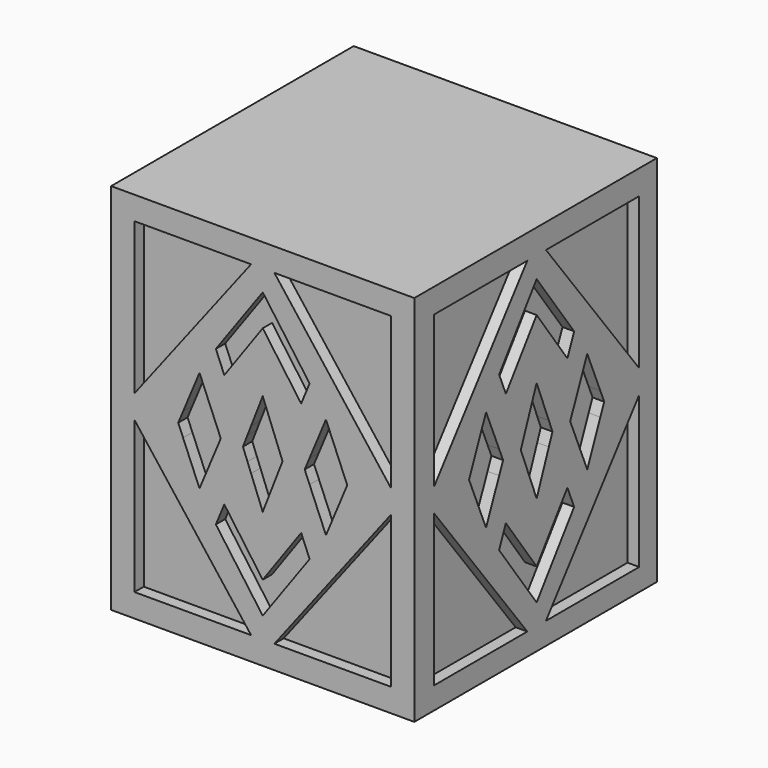
from build123d import *

# Parameters (mm, degrees)
F0_W     = 130
F0_H     = 130
F1_DEPTH = 160
F2_W     = 5
F2_H     = 5.0000008941
F2_H_2   = 5
F3_DEPTH = 5
F4_W     = 5
F4_H     = 5.0000008941
F4_H_2   = 5
F5_DEPTH = 5
F6_W     = 5
F6_H     = 5.0000008941
F6_H_2   = 5
F7_DEPTH = 5
F8_W     = 5
F8_H     = 5.0000008941
F8_H_2   = 5
F9_DEPTH = 5


# Not quite as in the source:
# - ends of sketch curves that miss each other by under 0.0002 mm in the source are joined


with BuildPart() as f1:
    # F0 (on Top) → F1 (new body)
    with BuildSketch(Plane.XY):
        with Locations((65, 65)):
            Rectangle(F0_W, F0_H)
    extrude(amount=F1_DEPTH)

    # F2 (on face) → F3 (cut)
    with BuildSketch(Plane.XZ):
        Polygon((85.1000148058, 113.1451874971), (65, 141.0418897867), (44.8999851942, 113.1451874971), (48.5190190375, 104.3991968036), (65, 127.470523119), (81.4809809625, 104.3991968036), align=None)
        Polygon((44.8999851942, 46.8548125029), (65, 18.9581102133), (85.1000148058, 46.8548125029), (81.4809809625, 55.6008031964), (65, 32.529476881), (48.5190190375, 55.6008031964), align=None)
        Polygon((120, 74.9999991059), (70, 10), (120, 10), align=None)
        Polygon((10, 74.999999702), (10, 10), (60, 10), align=None)
        Polygon((10, 150), (10, 85.0000008941), (60, 150), align=None)
        Polygon((120, 150), (70, 150), (120, 85.0000008941), align=None)
        Polygon((92.1118893847, 85.0000008941), (99.1458630462, 85.0000008941), (92.1118893847, 101.8357127905), align=None)
        Polygon((85.0779157232, 85.0000008941), (92.1118893847, 85.0000008941), (92.1118893847, 101.8357127905), align=None)
        Polygon((82.9889114201, 80), (92.1118893847, 80), (92.1118893847, 85.0000008941), (85.0779157232, 85.0000008941), align=None)
        Polygon((92.1118893847, 80), (101.2348673493, 80), (99.1458630462, 85.0000008941), (92.1118893847, 85.0000008941), align=None)
        Polygon((92.1118893847, 75), (99.1458634198, 75), (101.2348673493, 80), (92.1118893847, 80), align=None)
        Polygon((85.0779153496, 75), (92.1118893847, 75), (92.1118893847, 80), (82.9889114201, 80), align=None)
        Polygon((92.1118893847, 58.1642872095), (92.1118893847, 75), (85.0779153496, 75), align=None)
        Polygon((92.1118893847, 58.1642872095), (99.1458634198, 75), (92.1118893847, 75), align=None)
        Polygon((65, 101.8357127905), (65, 85.0000008941), (71.545128511, 85.0000008941), align=None)
        Polygon((60, 88.9744589067), (60, 85.0000008941), (65, 85.0000008941), (65, 101.8357127905), align=None)
        Polygon((60, 88.9744589067), (58.454871489, 85.0000008941), (60, 85.0000008941), align=None)
        Polygon((58.454871489, 85.0000008941), (56.5110482275, 80), (60, 80), (60, 85.0000008941), align=None)
        Polygon((56.5110482275, 80), (58.4548711414, 75), (60, 75), (60, 80), align=None)
        with Locations((62.5, 82.500000447)):
            Rectangle(F2_W, F2_H)
        with Locations((62.5, 77.5)):
            Rectangle(F2_W, F2_H_2)
        Polygon((65, 75), (60, 75), (60, 71.0255410933), (65, 58.1642872095), align=None)
        Polygon((71.5451288586, 75), (65, 75), (65, 58.1642872095), align=None)
        Polygon((65, 80), (65, 75), (71.5451288586, 75), (73.4889517725, 80), align=None)
        Polygon((65, 85.0000008941), (65, 80), (73.4889517725, 80), (71.545128511, 85.0000008941), align=None)
        Polygon((37.8881106153, 101.8357127905), (37.8881106153, 85.0000008941), (44.9220842768, 85.0000008941), align=None)
        Polygon((37.8881106153, 101.8357127905), (30.8541369538, 85.0000008941), (37.8881106153, 85.0000008941), align=None)
        Polygon((30.8541369538, 85.0000008941), (28.7651326507, 80), (37.8881106153, 80), (37.8881106153, 85.0000008941), align=None)
        Polygon((37.8881106153, 85.0000008941), (37.8881106153, 80), (47.0110885799, 80), (44.9220842768, 85.0000008941), align=None)
        Polygon((28.7651326507, 80), (30.8541365802, 75), (44.9220846504, 75), (47.0110885799, 80), (37.8881106153, 80), align=None)
        Polygon((44.9220846504, 75), (30.8541365802, 75), (37.8881106153, 58.1642872095), align=None)
        Polygon((60, 75), (58.4548711414, 75), (60, 71.0255410933), align=None)
    extrude(amount=-F3_DEPTH, mode=Mode.SUBTRACT)

    # F4 (on face) → F5 (cut)
    with BuildSketch(Plane.YZ.offset(130)):
        Polygon((85.6616547024, 112.6292116297), (65.5616398966, 140.5259139193), (45.4616250909, 112.6292116297), (49.0806589341, 103.8832209362), (65.5616398966, 126.9545472516), (82.0426208592, 103.8832209362), align=None)
        Polygon((85.6395556198, 84.4840250267), (92.6735292813, 84.4840250267), (92.6735292813, 101.3197369231), align=None)
        Polygon((92.6735292813, 84.4840250267), (99.7075029429, 84.4840250267), (92.6735292813, 101.3197369231), align=None)
        Polygon((92.6735292813, 79.4840241326), (101.7965072459, 79.4840241326), (99.7075029429, 84.4840250267), (92.6735292813, 84.4840250267), align=None)
        Polygon((83.5505513168, 79.4840241326), (92.6735292813, 79.4840241326), (92.6735292813, 84.4840250267), (85.6395556198, 84.4840250267), align=None)
        Polygon((85.6395552463, 74.4840241326), (92.6735292813, 74.4840241326), (92.6735292813, 79.4840241326), (83.5505513168, 79.4840241326), align=None)
        Polygon((92.6735292813, 74.4840241326), (99.7075033164, 74.4840241326), (101.7965072459, 79.4840241326), (92.6735292813, 79.4840241326), align=None)
        Polygon((92.6735292813, 57.6483113421), (99.7075033164, 74.4840241326), (92.6735292813, 74.4840241326), align=None)
        Polygon((92.6735292813, 57.6483113421), (92.6735292813, 74.4840241326), (85.6395552463, 74.4840241326), align=None)
        Polygon((65.5616398966, 101.3197369231), (65.5616398966, 84.4840250267), (72.1067684077, 84.4840250267), align=None)
        Polygon((60.5616398966, 88.4584830393), (60.5616398966, 84.4840250267), (65.5616398966, 84.4840250267), (65.5616398966, 101.3197369231), align=None)
        Polygon((60.5616398966, 88.4584830393), (59.0165113856, 84.4840250267), (60.5616398966, 84.4840250267), align=None)
        Polygon((59.0165113856, 84.4840250267), (57.0726881242, 79.4840241326), (60.5616398966, 79.4840241326), (60.5616398966, 84.4840250267), align=None)
        with Locations((63.0616398966, 81.9840245796)):
            Rectangle(F4_W, F4_H)
        Polygon((65.5616398966, 84.4840250267), (65.5616398966, 79.4840241326), (74.0505916691, 79.4840241326), (72.1067684077, 84.4840250267), align=None)
        Polygon((65.5616398966, 79.4840241326), (65.5616398966, 74.4840241326), (72.1067687553, 74.4840241326), (74.0505916691, 79.4840241326), align=None)
        with Locations((63.0616398966, 76.9840241326)):
            Rectangle(F4_W, F4_H_2)
        Polygon((57.0726881242, 79.4840241326), (59.016511038, 74.4840241326), (60.5616398966, 74.4840241326), (60.5616398966, 79.4840241326), align=None)
        Polygon((60.5616398966, 74.4840241326), (59.016511038, 74.4840241326), (60.5616398966, 70.5095652258), align=None)
        Polygon((65.5616398966, 74.4840241326), (60.5616398966, 74.4840241326), (60.5616398966, 70.5095652258), (65.5616398966, 57.6483113421), align=None)
        Polygon((72.1067687553, 74.4840241326), (65.5616398966, 74.4840241326), (65.5616398966, 57.6483113421), align=None)
        Polygon((38.449750512, 101.3197369231), (38.449750512, 84.4840250267), (45.4837241735, 84.4840250267), align=None)
        Polygon((38.449750512, 101.3197369231), (31.4157768504, 84.4840250267), (38.449750512, 84.4840250267), align=None)
        Polygon((31.4157768504, 84.4840250267), (29.3267725474, 79.4840241326), (38.449750512, 79.4840241326), (38.449750512, 84.4840250267), align=None)
        Polygon((38.449750512, 84.4840250267), (38.449750512, 79.4840241326), (47.5727284765, 79.4840241326), (45.4837241735, 84.4840250267), align=None)
        Polygon((29.3267725474, 79.4840241326), (31.4157764769, 74.4840241326), (45.483724547, 74.4840241326), (47.5727284765, 79.4840241326), (38.449750512, 79.4840241326), align=None)
        Polygon((45.483724547, 74.4840241326), (31.4157764769, 74.4840241326), (38.449750512, 57.6483113421), align=None)
        Polygon((45.4616250909, 46.3388366354), (65.5616398966, 18.4421343459), (85.6616547024, 46.3388366354), (82.0426208592, 55.084827329), (65.5616398966, 32.0135010136), (49.0806589341, 55.084827329), align=None)
        Polygon((10.5616398966, 74.4840238346), (10.5616398966, 9.4840241326), (60.5616398966, 9.4840241326), align=None)
        Polygon((120.5616398966, 74.4840232385), (70.5616398966, 9.4840241326), (120.5616398966, 9.4840241326), align=None)
        Polygon((120.5616398966, 149.4840241326), (70.5616398966, 149.4840241326), (120.5616398966, 84.4840250267), align=None)
        Polygon((10.5616398966, 149.4840241326), (10.5616398966, 84.4840250267), (60.5616398966, 149.4840241326), align=None)
    extrude(amount=-F5_DEPTH, mode=Mode.SUBTRACT)

    # F6 (on face) → F7 (cut)
    with BuildSketch(Plane(origin=(0, 130, 0), x_dir=(-1, 0, 0), z_dir=(0, 1, 0))):
        Polygon((-119.4383601034, 149.4840241326), (-119.4383601034, 84.4840250267), (-69.4383601034, 149.4840241326), align=None)
        Polygon((-9.4383601034, 149.4840241326), (-59.4383601034, 149.4840241326), (-9.4383601034, 84.4840250267), align=None)
        Polygon((-44.3383452976, 112.6292116297), (-64.4383601034, 140.5259139193), (-84.5383749091, 112.6292116297), (-80.9193410659, 103.8832209362), (-64.4383601034, 126.9545472516), (-47.9573791408, 103.8832209362), align=None)
        Polygon((-37.3264707187, 84.4840250267), (-30.2924970571, 84.4840250267), (-37.3264707187, 101.3197369231), align=None)
        Polygon((-44.3604443802, 84.4840250267), (-37.3264707187, 84.4840250267), (-37.3264707187, 101.3197369231), align=None)
        Polygon((-46.4494486832, 79.4840241326), (-37.3264707187, 79.4840241326), (-37.3264707187, 84.4840250267), (-44.3604443802, 84.4840250267), align=None)
        Polygon((-37.3264707187, 79.4840241326), (-28.2034927541, 79.4840241326), (-30.2924970571, 84.4840250267), (-37.3264707187, 84.4840250267), align=None)
        Polygon((-37.3264707187, 74.4840241326), (-30.2924966836, 74.4840241326), (-28.2034927541, 79.4840241326), (-37.3264707187, 79.4840241326), align=None)
        Polygon((-44.3604447537, 74.4840241326), (-37.3264707187, 74.4840241326), (-37.3264707187, 79.4840241326), (-46.4494486832, 79.4840241326), align=None)
        Polygon((-37.3264707187, 57.6483113421), (-37.3264707187, 74.4840241326), (-44.3604447537, 74.4840241326), align=None)
        Polygon((-37.3264707187, 57.6483113421), (-30.2924966836, 74.4840241326), (-37.3264707187, 74.4840241326), align=None)
        Polygon((-64.4383601034, 101.3197369231), (-64.4383601034, 84.4840250267), (-57.8932315923, 84.4840250267), align=None)
        Polygon((-69.4383601034, 88.4584830393), (-69.4383601034, 84.4840250267), (-64.4383601034, 84.4840250267), (-64.4383601034, 101.3197369231), align=None)
        Polygon((-69.4383601034, 88.4584830393), (-70.9834886144, 84.4840250267), (-69.4383601034, 84.4840250267), align=None)
        Polygon((-70.9834886144, 84.4840250267), (-72.9273118758, 79.4840241326), (-69.4383601034, 79.4840241326), (-69.4383601034, 84.4840250267), align=None)
        with Locations((-66.9383601034, 81.9840245796)):
            Rectangle(F6_W, F6_H)
        Polygon((-64.4383601034, 84.4840250267), (-64.4383601034, 79.4840241326), (-55.9494083309, 79.4840241326), (-57.8932315923, 84.4840250267), align=None)
        Polygon((-64.4383601034, 79.4840241326), (-64.4383601034, 74.4840241326), (-57.8932312447, 74.4840241326), (-55.9494083309, 79.4840241326), align=None)
        with Locations((-66.9383601034, 76.9840241326)):
            Rectangle(F6_W, F6_H_2)
        Polygon((-72.9273118758, 79.4840241326), (-70.983488962, 74.4840241326), (-69.4383601034, 74.4840241326), (-69.4383601034, 79.4840241326), align=None)
        Polygon((-69.4383601034, 74.4840241326), (-70.983488962, 74.4840241326), (-69.4383601034, 70.5095652258), align=None)
        Polygon((-64.4383601034, 74.4840241326), (-69.4383601034, 74.4840241326), (-69.4383601034, 70.5095652258), (-64.4383601034, 57.6483113421), align=None)
        Polygon((-57.8932312447, 74.4840241326), (-64.4383601034, 74.4840241326), (-64.4383601034, 57.6483113421), align=None)
        Polygon((-91.550249488, 101.3197369231), (-91.550249488, 84.4840250267), (-84.5162758265, 84.4840250267), align=None)
        Polygon((-91.550249488, 101.3197369231), (-98.5842231496, 84.4840250267), (-91.550249488, 84.4840250267), align=None)
        Polygon((-98.5842231496, 84.4840250267), (-100.6732274526, 79.4840241326), (-91.550249488, 79.4840241326), (-91.550249488, 84.4840250267), align=None)
        Polygon((-91.550249488, 84.4840250267), (-91.550249488, 79.4840241326), (-82.4272715235, 79.4840241326), (-84.5162758265, 84.4840250267), align=None)
        Polygon((-100.6732274526, 79.4840241326), (-98.5842235231, 74.4840241326), (-84.516275453, 74.4840241326), (-82.4272715235, 79.4840241326), (-91.550249488, 79.4840241326), align=None)
        Polygon((-84.516275453, 74.4840241326), (-98.5842235231, 74.4840241326), (-91.550249488, 57.6483113421), align=None)
        Polygon((-84.5383749091, 46.3388366354), (-64.4383601034, 18.4421343459), (-44.3383452976, 46.3388366354), (-47.9573791408, 55.084827329), (-64.4383601034, 32.0135010136), (-80.9193410659, 55.084827329), align=None)
        Polygon((-119.4383601034, 74.4840238346), (-119.4383601034, 9.4840241326), (-69.4383601034, 9.4840241326), align=None)
        Polygon((-9.4383601034, 74.4840232385), (-59.4383601034, 9.4840241326), (-9.4383601034, 9.4840241326), align=None)
    extrude(amount=-F7_DEPTH, mode=Mode.SUBTRACT)

    # F8 (on face) → F9 (cut)
    with BuildSketch(Plane(origin=(0, 0, 0), x_dir=(0, -1, 0), z_dir=(-1, 0, 0))):
        Polygon((-9.4383601034, 149.4840241326), (-59.4383601034, 149.4840241326), (-9.4383601034, 84.4840250267), align=None)
        Polygon((-44.3383452976, 112.6292116297), (-64.4383601034, 140.5259139193), (-84.5383749091, 112.6292116297), (-80.9193410659, 103.8832209362), (-64.4383601034, 126.9545472516), (-47.9573791408, 103.8832209362), align=None)
        Polygon((-119.4383601034, 149.4840241326), (-119.4383601034, 84.4840250267), (-69.4383601034, 149.4840241326), align=None)
        Polygon((-37.3264707187, 84.4840250267), (-30.2924970571, 84.4840250267), (-37.3264707187, 101.3197369231), align=None)
        Polygon((-44.3604443802, 84.4840250267), (-37.3264707187, 84.4840250267), (-37.3264707187, 101.3197369231), align=None)
        Polygon((-46.4494486832, 79.4840241326), (-37.3264707187, 79.4840241326), (-37.3264707187, 84.4840250267), (-44.3604443802, 84.4840250267), align=None)
        Polygon((-37.3264707187, 79.4840241326), (-28.2034927541, 79.4840241326), (-30.2924970571, 84.4840250267), (-37.3264707187, 84.4840250267), align=None)
        Polygon((-37.3264707187, 74.4840241326), (-30.2924966836, 74.4840241326), (-28.2034927541, 79.4840241326), (-37.3264707187, 79.4840241326), align=None)
        Polygon((-37.3264707187, 57.6483113421), (-30.2924966836, 74.4840241326), (-37.3264707187, 74.4840241326), align=None)
        Polygon((-37.3264707187, 57.6483113421), (-37.3264707187, 74.4840241326), (-44.3604447537, 74.4840241326), align=None)
        Polygon((-44.3604447537, 74.4840241326), (-37.3264707187, 74.4840241326), (-37.3264707187, 79.4840241326), (-46.4494486832, 79.4840241326), align=None)
        Polygon((-64.4383601034, 101.3197369231), (-64.4383601034, 84.4840250267), (-57.8932315923, 84.4840250267), align=None)
        Polygon((-69.4383601034, 88.4584830393), (-69.4383601034, 84.4840250267), (-64.4383601034, 84.4840250267), (-64.4383601034, 101.3197369231), align=None)
        Polygon((-69.4383601034, 88.4584830393), (-70.9834886144, 84.4840250267), (-69.4383601034, 84.4840250267), align=None)
        Polygon((-70.9834886144, 84.4840250267), (-72.9273118758, 79.4840241326), (-69.4383601034, 79.4840241326), (-69.4383601034, 84.4840250267), align=None)
        with Locations((-66.9383601034, 81.9840245796)):
            Rectangle(F8_W, F8_H)
        Polygon((-64.4383601034, 84.4840250267), (-64.4383601034, 79.4840241326), (-55.9494083309, 79.4840241326), (-57.8932315923, 84.4840250267), align=None)
        Polygon((-64.4383601034, 79.4840241326), (-64.4383601034, 74.4840241326), (-57.8932312447, 74.4840241326), (-55.9494083309, 79.4840241326), align=None)
        with Locations((-66.9383601034, 76.9840241326)):
            Rectangle(F8_W, F8_H_2)
        Polygon((-72.9273118758, 79.4840241326), (-70.983488962, 74.4840241326), (-69.4383601034, 74.4840241326), (-69.4383601034, 79.4840241326), align=None)
        Polygon((-69.4383601034, 74.4840241326), (-70.983488962, 74.4840241326), (-69.4383601034, 70.5095652258), align=None)
        Polygon((-64.4383601034, 74.4840241326), (-69.4383601034, 74.4840241326), (-69.4383601034, 70.5095652258), (-64.4383601034, 57.6483113421), align=None)
        Polygon((-57.8932312447, 74.4840241326), (-64.4383601034, 74.4840241326), (-64.4383601034, 57.6483113421), align=None)
        Polygon((-84.516275453, 74.4840241326), (-98.5842235231, 74.4840241326), (-91.550249488, 57.6483113421), align=None)
        Polygon((-100.6732274526, 79.4840241326), (-98.5842235231, 74.4840241326), (-84.516275453, 74.4840241326), (-82.4272715235, 79.4840241326), (-91.550249488, 79.4840241326), align=None)
        Polygon((-91.550249488, 84.4840250267), (-91.550249488, 79.4840241326), (-82.4272715235, 79.4840241326), (-84.5162758265, 84.4840250267), align=None)
        Polygon((-98.5842231496, 84.4840250267), (-100.6732274526, 79.4840241326), (-91.550249488, 79.4840241326), (-91.550249488, 84.4840250267), align=None)
        Polygon((-91.550249488, 101.3197369231), (-98.5842231496, 84.4840250267), (-91.550249488, 84.4840250267), align=None)
        Polygon((-91.550249488, 101.3197369231), (-91.550249488, 84.4840250267), (-84.5162758265, 84.4840250267), align=None)
        Polygon((-84.5383749091, 46.3388366354), (-64.4383601034, 18.4421343459), (-44.3383452976, 46.3388366354), (-47.9573791408, 55.084827329), (-64.4383601034, 32.0135010136), (-80.9193410659, 55.084827329), align=None)
        Polygon((-9.4383601034, 74.4840232385), (-59.4383601034, 9.4840241326), (-9.4383601034, 9.4840241326), align=None)
        Polygon((-119.4383601034, 74.4840238346), (-119.4383601034, 9.4840241326), (-69.4383601034, 9.4840241326), align=None)
    extrude(amount=-F9_DEPTH, mode=Mode.SUBTRACT)


solid = f1.part
